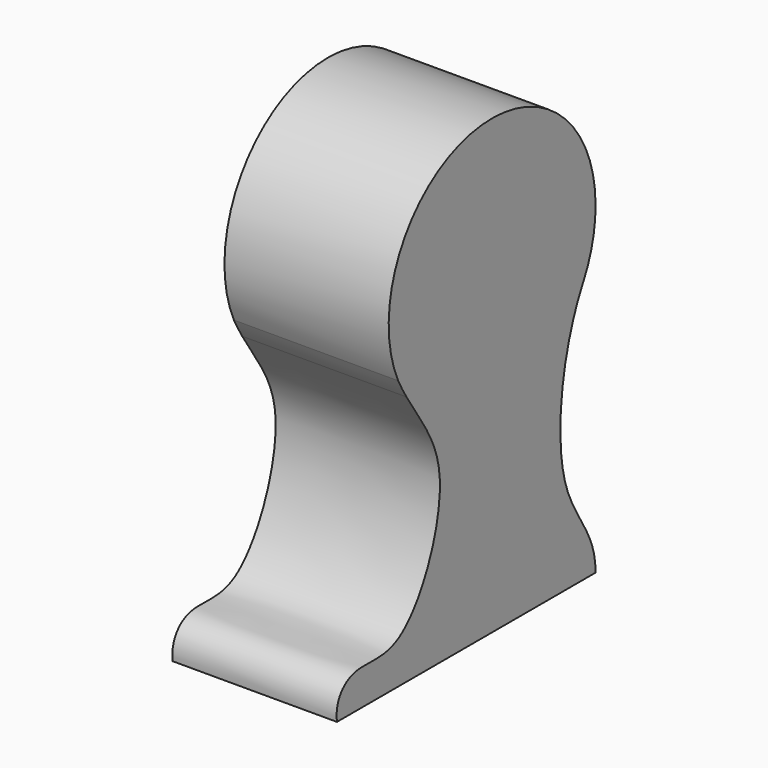
from build123d import *

# Parameters (mm, degrees)
F1_DEPTH = 12.7


# Not quite as in the source:
# - a feature names something its author has since deleted; it is built from what else it names


with BuildPart() as f1:
    # F0 (on Right) → F1 (new body)
    with BuildSketch(Plane.YZ):
        with BuildLine():
            Line((-25, 0), (0, 0))
            add(Edge.make_bspline(
                [(0, 0), (0, 2.8664874844), (-4.4847679358, 6.1521378453), (-3.3497820964, 16.197657633), (-1.2690202208, 20.1245521133)],
                knots=[0, 0, 0, 0, 0.4275233277, 0.9891624175, 0.9891624175, 0.9891624175, 0.9891624175], degree=3))
            ThreePointArc((-1.2690202208, 20.1245521133), (-9.5726785605, 15.0091343525), (-18.2827975356, 19.3968522253))
            add(Edge.make_bspline(
                [(-25, 0), (-25.2065360546, 1.3745123288), (-23.5834985534, 3.4868467231), (-18.1413165506, 1.4671690224), (-13.2206567534, 12.9916001305), (-16.9008347887, 17.1648896009), (-18.2827975356, 19.3968522253)],
                knots=[0, 0, 0, 0, 0.1737603194, 0.3817412709, 0.7004550662, 0.949115937, 0.949115937, 0.949115937, 0.949115937], degree=3))
        make_face()
        with BuildLine():
            ThreePointArc((-18.2827975356, 19.3968522253), (-9.5726785605, 15.0091343525), (-1.2690202208, 20.1245521133))
            add(Edge.make_bspline(
                [(-1.2690202208, 20.1245521133), (-1.2288691187, 20.2003268299), (-1.1881832022, 20.2754399281), (-1.1469651688, 20.3498629828)],
                knots=[0.9891624175, 0.9891624175, 0.9891624175, 0.9891624175, 1, 1, 1, 1], degree=3))
            ThreePointArc((-1.1469651688, 20.3498629828), (-0.2909746032, 22.6052503588), (0, 25))
            ThreePointArc((0, 25), (-12.1351726564, 34.7693929047), (-19.0882075454, 20.82813188))
            add(Edge.make_bspline(
                [(-18.2827975356, 19.3968522253), (-18.5655918459, 19.853584024), (-18.8387159675, 20.3271892353), (-19.0882075454, 20.82813188)],
                knots=[0.949115937, 0.949115937, 0.949115937, 0.949115937, 1, 1, 1, 1], degree=3))
        make_face()
    extrude(amount=F1_DEPTH)


solid = f1.part
